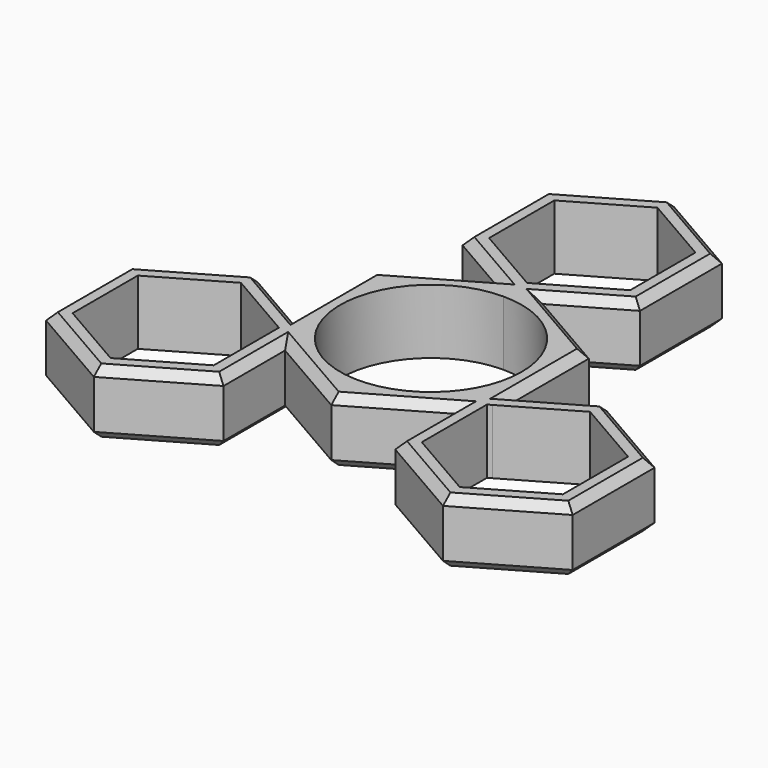
from build123d import *

# Parameters (mm, degrees)
F1_DEPTH = 8
F2_SIZE  = 1


# Not quite as in the source:
# - a feature names something its author has since deleted; it is built from what else it names


with BuildPart() as f1:
    # F0 (on Top) → F1 (new body)
    with BuildSketch(Plane.XY):
        Polygon((2.7355143452, 13.8776440214), (0, 12.2982940778), (-2.7355143452, 13.8776440214), (-13.3861494398, 7.7284969825), (-13.3861494398, -4.5697970953), (-10.6506350946, -6.1491470389), (-10.6506350946, -9.3078469261), (0, -15.456993965), (10.6506350946, -9.3078469261), (10.6506350946, -6.1491470389), (13.3861494398, -4.5697970953), (13.3861494398, 7.7284969825), align=None)
        with BuildLine():
            ThreePointArc((0, 11.25), (7.9549512883, 7.9549512883), (11.25, 0))
            ThreePointArc((11.25, 0), (-7.9549512883, -7.9549512883), (0, 11.25))
        make_face(mode=Mode.SUBTRACT)
        Polygon((-2.7355143452, 13.8776440214), (0, 12.2982940778), (0, 14.8963702892), (-0.4855143452, 15.1766821271), align=None)
        Polygon((0, 14.8963702892), (0, 12.2982940778), (2.7355143452, 13.8776440214), (0.4855143452, 15.1766821271), align=None)
        Polygon((-11, 18.6491470389), (-2.7355143452, 13.8776440214), (-0.4855143452, 15.1766821271), (-8.75, 19.9481851446), (-8.75, 30.0518148554), (0, 35.1036297108), (8.75, 30.0518148554), (8.75, 19.9481851446), (0.4855143452, 15.1766821271), (2.7355143452, 13.8776440214), (11, 18.6491470389), (11, 31.3508529611), (0, 37.7017059222), (-11, 31.3508529611), align=None)
        Polygon((-13.3861494398, -7.1678733067), (-13.3861494398, -4.5697970953), (-21.6506350946, 0.2017059222), (-32.6506350946, -6.1491470389), (-32.6506350946, -18.8508529611), (-21.6506350946, -25.2017059222), (-10.6506350946, -18.8508529611), (-10.6506350946, -9.3078469261), (-12.9006350946, -8.0088088204), (-12.9006350946, -17.5518148554), (-21.6506350946, -22.6036297108), (-30.4006350946, -17.5518148554), (-30.4006350946, -7.4481851446), (-21.6506350946, -2.3963702892), align=None)
        Polygon((-10.6506350946, -6.1491470389), (-13.3861494398, -4.5697970953), (-13.3861494398, -7.1678733067), (-12.9006350946, -7.4481851446), (-12.9006350946, -8.0088088204), (-10.6506350946, -9.3078469261), align=None)
        Polygon((13.3861494398, -7.1678733067), (13.3861494398, -4.5697970953), (10.6506350946, -6.1491470389), (10.6506350946, -9.3078469261), (12.9006350946, -8.0088088204), (12.9006350946, -7.4481851446), align=None)
        Polygon((21.6506350946, 0.2017059222), (13.3861494398, -4.5697970953), (13.3861494398, -7.1678733067), (21.6506350946, -2.3963702892), (30.4006350946, -7.4481851446), (30.4006350946, -17.5518148554), (21.6506350946, -22.6036297108), (12.9006350946, -17.5518148554), (12.9006350946, -8.0088088204), (10.6506350946, -9.3078469261), (10.6506350946, -18.8508529611), (21.6506350946, -25.2017059222), (32.6506350946, -18.8508529611), (32.6506350946, -6.1491470389), align=None)
    extrude(amount=F1_DEPTH)

    # F2
    f2_edges = [f1.edges().sort_by_distance(p)[0] for p in [
        (-8.060832, 10.803071, 8),
        (-13.386149, 1.57935, 8),
        (-17.518392, -2.184046, 8),
        (-27.150635, -2.973721, 8),
        (-32.650635, -12.5, 8),
        (-27.150635, -22.026279, 8),
        (-16.150635, -22.026279, 8),
        (-5.325318, -12.38242, 8),
        (-10.650635, -14.07935, 8),
        (5.325318, -12.38242, 8),
        (10.650635, -14.07935, 8),
        (16.150635, -22.026279, 8),
        (27.150635, -22.026279, 8),
        (32.650635, -12.5, 8),
        (27.150635, -2.973721, 8),
        (17.518392, -2.184046, 8),
        (13.386149, 1.57935, 8),
        (8.060832, 10.803071, 8),
        (6.867757, 16.263396, 8),
        (11, 25, 8),
        (5.5, 34.526279, 8),
        (-5.5, 34.526279, 8),
        (-11, 25, 8),
        (-6.867757, 16.263396, 8),
        (-11, 25, 0),
        (-5.5, 34.526279, 0),
        (5.5, 34.526279, 0),
        (11, 25, 0),
        (6.867757, 16.263396, 0),
        (-6.867757, 16.263396, 0),
        (-8.060832, 10.803071, 0),
        (8.060832, 10.803071, 0),
        (13.386149, 1.57935, 0),
        (-13.386149, 1.57935, 0),
        (17.518392, -2.184046, 0),
        (27.150635, -2.973721, 0),
        (32.650635, -12.5, 0),
        (27.150635, -22.026279, 0),
        (16.150635, -22.026279, 0),
        (10.650635, -14.07935, 0),
        (5.325318, -12.38242, 0),
        (-5.325318, -12.38242, 0),
        (-10.650635, -14.07935, 0),
        (-16.150635, -22.026279, 0),
        (-27.150635, -22.026279, 0),
        (-32.650635, -12.5, 0),
        (-27.150635, -2.973721, 0),
        (-17.518392, -2.184046, 0),
    ]]
    chamfer(f2_edges, length=F2_SIZE)


solid = f1.part
